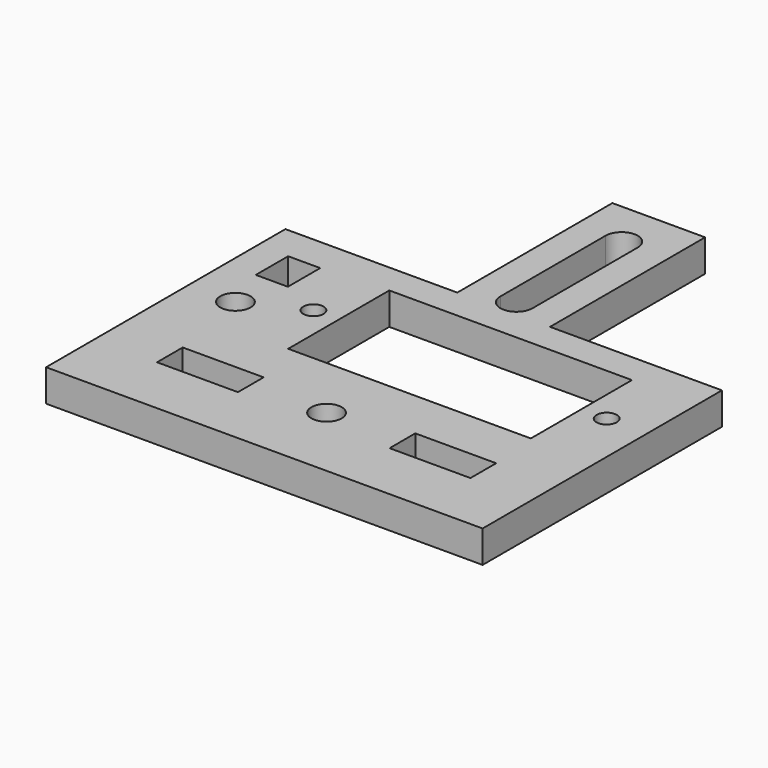
from build123d import *

# Parameters (mm, degrees)
F0_W     = 8
F0_H     = 3.175
F0_R     = 1.5
F0_W_2   = 3.175
F0_H_2   = 4
F0_R_2   = 1
F0_W_3   = 24
F0_H_3   = 12.5
F1_DEPTH = 3.175


# Not quite as in the source:
# - a length typed as a fraction of an inch, garbled in the dataset ("3 / 203.2 mm" for 3/8 in), is restored


with BuildPart() as f1:
    # F0 (on Top) → F1 (new body)
    with BuildSketch(Plane.XY):
        Polygon((-34.1063038088, 0.9337500209), (-34.1063038088, -28.6537499791), (9.0686961912, -28.6537499791), (9.0686961912, 0.9337500209), (-7.9313038088, 0.9337500209), (-7.9313038088, 20.1087500209), (-17.1063038088, 20.1087500209), (-17.1063038088, 0.9337500209), align=None)
        with Locations((-23.9313038088, -21.0662499791)):
            Rectangle(F0_W, F0_H, mode=Mode.SUBTRACT)
        with Locations((-29.5188038088, -10.9787499791)):
            Circle(F0_R, mode=Mode.SUBTRACT)
        with Locations((-29.5188038088, -4.4787499791)):
            Rectangle(F0_W_2, F0_H_2, mode=Mode.SUBTRACT)
        with Locations((-23.9313038088, -8.3162499791)):
            Circle(F0_R_2, mode=Mode.SUBTRACT)
        with Locations((-12.4313038088, -21.0662499791)):
            Circle(F0_R, mode=Mode.SUBTRACT)
        with Locations((-0.9313038088, -21.0662499791)):
            Rectangle(F0_W, F0_H, mode=Mode.SUBTRACT)
        with Locations((-9.4313038088, -8.3162499791)):
            Rectangle(F0_W_3, F0_H_3, mode=Mode.SUBTRACT)
        with Locations((5.0686961912, -8.3162499791)):
            Circle(F0_R_2, mode=Mode.SUBTRACT)
        with BuildLine():
            ThreePointArc((-14.1063038088, 15.5212500209), (-12.5188038088, 17.1087500209), (-10.9313038088, 15.5212500209))
            Line((-10.9313038088, 15.5212500209), (-10.9313038088, 2.5212500209))
            ThreePointArc((-10.9313038088, 2.5212500209), (-12.5188038088, 0.9337500209), (-14.1063038088, 2.5212500209))
            Line((-14.1063038088, 2.5212500209), (-14.1063038088, 15.5212500209))
        make_face(mode=Mode.SUBTRACT)
    extrude(amount=F1_DEPTH)


solid = f1.part
